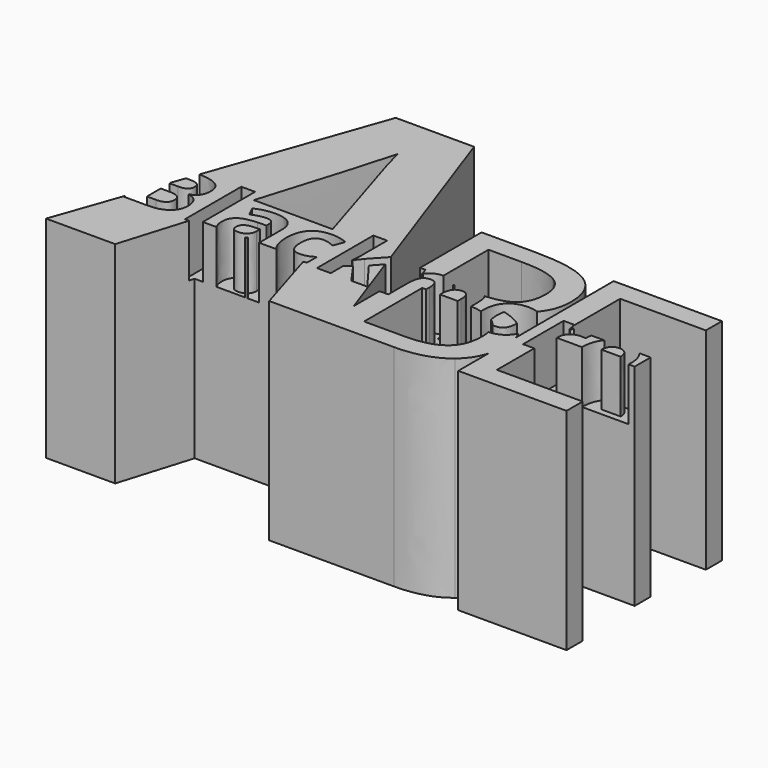
from build123d import *

# Parameters (mm, degrees)
F1_DEPTH     = 20
F2_TEXT_SIZE = 8.807554657
F3_DEPTH     = 5


# Not quite as in the source:
# - Text() gives the source's letters only with a copy of the font that has no kerning and outlines rounded to 1/6400 em; it was checked with that copy


with BuildPart() as f1:
    # F0 (on Top) → F1 (new body)
    with BuildSketch(Plane.XY):
        Polygon((-39.3541229361, -15.4000898603), (-37.2749521763, -22.2343429923), (-31.8759119989, -22.2343429923), (-31.8759119989, -18.9504013195), (-40.8868047047, 6.5850994429), (-48.3240801719, 6.5850994429), (-58.4561116993, -22.2343429923), (-51.8982438043, -22.2343429923), (-49.8190730445, -15.4000898603), align=None)
        with BuildLine():
            add(Edge.make_bspline(
                [(-40.8114269128, -10.299525942), (-43.6946274529, -1.0154945733), (-44.058953447, 0.2031130623)],
                knots=[0, 0, 0, 1, 1, 1], degree=2))
            Line((-40.8114269128, -10.299525942), (-48.2863912759, -10.299525942))
            add(Edge.make_bspline(
                [(-44.5803165077, 2.1252467557), (-45.2273092214, -0.3873463075), (-48.2863912759, -10.299525942)],
                knots=[0, 0, 0, 1, 1, 1], degree=2))
            add(Edge.make_bspline(
                [(-44.058953447, 0.2031130623), (-44.4232794412, 1.421720698), (-44.5803165077, 2.1252467557)],
                knots=[0, 0, 0, 1, 1, 1], degree=2))
        make_face(mode=Mode.SUBTRACT)
        Polygon((-31.8759119989, -18.9504013195), (-31.8759119989, -22.2343429923), (-30.7170842813, -22.2343429923), align=None)
        with BuildLine():
            Line((-31.8759119989, -18.9504013195), (-30.7170842813, -22.2343429923))
            Line((-30.7170842813, -22.2343429923), (-25.4431825327, -22.2343429923))
            add(Edge.make_bspline(
                [(-20.7699700346, -20.8461002468), (-22.4407040365, -22.2343429923), (-25.4431825327, -22.2343429923)],
                knots=[0, 0, 0, 1, 1, 1], degree=2))
            add(Edge.make_bspline(
                [(-19.3340054438, -18.6877359219), (-19.7255244947, -19.9782517788), (-20.7699700346, -20.8461002468)],
                knots=[0.3748582726, 0.3748582726, 0.3748582726, 1, 1, 1], degree=2))
            Line((-19.3340054438, -18.6877359219), (-19.3340054438, -15.4067827387))
            add(Edge.make_bspline(
                [(-23.3002845737, -12.5731420248), (-20.092351178, -13.1216647381), (-19.3340054438, -15.4067827387)],
                knots=[0, 0, 0, 0.7636030302, 0.7636030302, 0.7636030302], degree=2))
            Line((-23.3002845737, -12.5731420248), (-23.3002845737, -12.4480387542))
            add(Edge.make_bspline(
                [(-20.6307422011, -11.0678671874), (-21.5448031949, -12.1332627828), (-23.3002845737, -12.4480387542)],
                knots=[0, 0, 0, 1, 1, 1], degree=2))
            add(Edge.make_bspline(
                [(-19.7166812073, -8.3599867157), (-19.7166812073, -10.002471592), (-20.6307422011, -11.0678671874)],
                knots=[0, 0, 0, 1, 1, 1], degree=2))
            add(Edge.make_bspline(
                [(-21.3571482889, -4.8934154413), (-19.7166812073, -5.9910957517), (-19.7166812073, -8.3599867157)],
                knots=[0, 0, 0, 1, 1, 1], degree=2))
            add(Edge.make_bspline(
                [(-26.6659661137, -3.7957351309), (-22.9976153705, -3.7957351309), (-21.3571482889, -4.8934154413)],
                knots=[0, 0, 0, 1, 1, 1], degree=2))
            Line((-26.6659661137, -3.7957351309), (-31.8759119989, -3.7957351309))
            Line((-31.8759119989, -3.7957351309), (-31.8759119989, -18.9504013195))
        make_face()
        with BuildLine():
            Line((-29.7330140399, -20.4062210047), (-29.7330140399, -13.5053631708))
            Line((-29.7330140399, -13.5053631708), (-26.0606277073, -13.5053631708))
            add(Edge.make_bspline(
                [(-22.5496649497, -14.3124810461), (-23.7038435114, -13.5053631708), (-26.0606277073, -13.5053631708)],
                knots=[0, 0, 0, 1, 1, 1], degree=2))
            add(Edge.make_bspline(
                [(-21.395486388, -16.8347244065), (-21.395486388, -15.1195989215), (-22.5496649497, -14.3124810461)],
                knots=[0, 0, 0, 1, 1, 1], degree=2))
            add(Edge.make_bspline(
                [(-22.5234336187, -19.5426048781), (-21.395486388, -18.6789887516), (-21.395486388, -16.8347244065)],
                knots=[0, 0, 0, 1, 1, 1], degree=2))
            add(Edge.make_bspline(
                [(-25.8830617747, -20.4062210047), (-23.6513808495, -20.4062210047), (-22.5234336187, -19.5426048781)],
                knots=[0, 0, 0, 1, 1, 1], degree=2))
            Line((-25.8830617747, -20.4062210047), (-29.7330140399, -20.4062210047))
        make_face(mode=Mode.SUBTRACT)
        with BuildLine():
            Line((-26.2018733354, -11.6893479514), (-29.7330140399, -11.6893479514))
            Line((-29.7330140399, -11.6893479514), (-29.7330140399, -5.6521062441))
            Line((-29.7330140399, -5.6521062441), (-26.5771831475, -5.6521062441))
            add(Edge.make_bspline(
                [(-23.046042443, -6.3381564381), (-24.1558295215, -5.6521062441), (-26.5771831475, -5.6521062441)],
                knots=[0, 0, 0, 1, 1, 1], degree=2))
            add(Edge.make_bspline(
                [(-21.9362553644, -8.5779085421), (-21.9362553644, -7.0242066321), (-23.046042443, -6.3381564381)],
                knots=[0, 0, 0, 1, 1, 1], degree=2))
            add(Edge.make_bspline(
                [(-22.9330459404, -10.9770664264), (-21.9362553644, -10.2647849015), (-21.9362553644, -8.5779085421)],
                knots=[0, 0, 0, 1, 1, 1], degree=2))
            add(Edge.make_bspline(
                [(-26.2018733354, -11.6893479514), (-23.9298365164, -11.6893479514), (-22.9330459404, -10.9770664264)],
                knots=[0, 0, 0, 1, 1, 1], degree=2))
        make_face(mode=Mode.SUBTRACT)
        with BuildLine():
            Line((-19.3340054438, -15.4067827387), (-19.3340054438, -18.6877359219))
            add(Edge.make_bspline(
                [(-19.0992360327, -16.9880768028), (-19.0992360327, -17.9138945292), (-19.3340054438, -18.6877359219)],
                knots=[0, 0, 0, 0.3748582726, 0.3748582726, 0.3748582726], degree=2))
            add(Edge.make_bspline(
                [(-19.3340054438, -15.4067827387), (-19.0992360327, -16.1142117951), (-19.0992360327, -16.9880768028)],
                knots=[0.7636030302, 0.7636030302, 0.7636030302, 1, 1, 1], degree=2))
        make_face()
        with BuildLine():
            add(Edge.make_bspline(
                [(-19.0992360327, -16.9880768028), (-19.0992360327, -17.9138945292), (-19.3340054438, -18.6877359219)],
                knots=[0, 0, 0, 0.3748582726, 0.3748582726, 0.3748582726], degree=2))
            Line((-19.3340054438, -18.6877359219), (-19.3340054438, -22.2343429923))
            Line((-19.3340054438, -22.2343429923), (-9.0553593017, -22.2343429923))
            Line((-9.0553593017, -22.2343429923), (-9.0553593017, -20.3174380384))
            Line((-9.0553593017, -20.3174380384), (-17.1911074848, -20.3174380384))
            Line((-17.1911074848, -20.3174380384), (-17.1911074848, -13.5336122965))
            Line((-17.1911074848, -13.5336122965), (-9.5477012056, -13.5336122965))
            Line((-9.5477012056, -13.5336122965), (-9.5477012056, -11.6409208789))
            Line((-9.5477012056, -11.6409208789), (-17.1911074848, -11.6409208789))
            Line((-17.1911074848, -11.6409208789), (-17.1911074848, -5.7005333166))
            Line((-17.1911074848, -5.7005333166), (-9.0553593017, -5.7005333166))
            Line((-9.0553593017, -5.7005333166), (-9.0553593017, -3.7957351309))
            Line((-9.0553593017, -3.7957351309), (-19.3340054438, -3.7957351309))
            Line((-19.3340054438, -3.7957351309), (-19.3340054438, -15.4067827387))
            add(Edge.make_bspline(
                [(-19.3340054438, -15.4067827387), (-19.0992360327, -16.1142117951), (-19.0992360327, -16.9880768028)],
                knots=[0.7636030302, 0.7636030302, 0.7636030302, 1, 1, 1], degree=2))
        make_face()
    extrude(amount=F1_DEPTH)

    # F2 (on face) → F3 (cut)
    with BuildSketch(Plane.XY.offset(20)):
        with Locations((-56.9612458348, -15.8929036393)):
            Text('Blackmore', F2_TEXT_SIZE, font='Open Sans', font_style=FontStyle.BOLD, text_align=(TextAlign.LEFT, TextAlign.BOTTOM))
    extrude(amount=-F3_DEPTH, mode=Mode.SUBTRACT)


solid = f1.part
